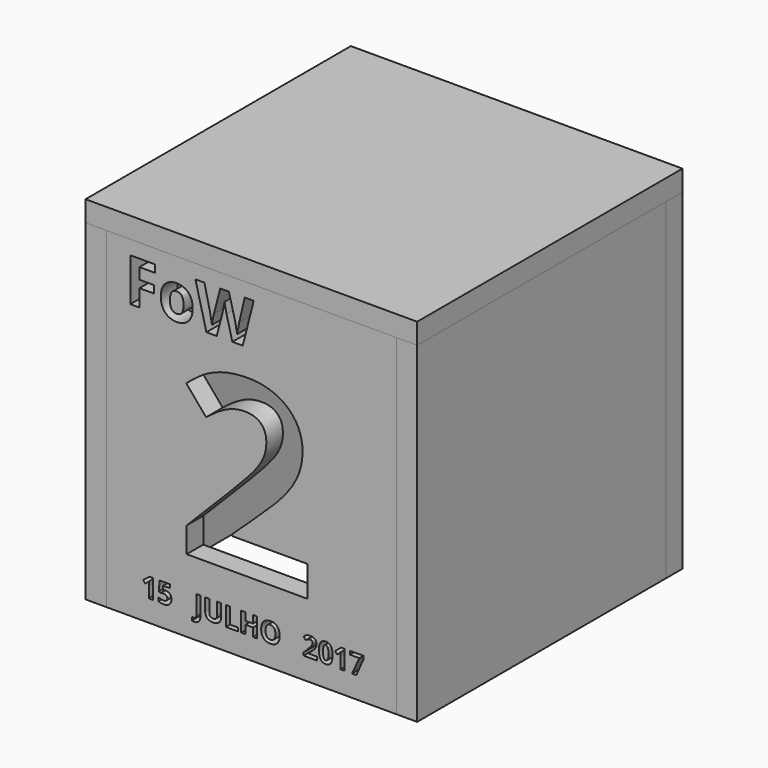
from build123d import *

# Parameters (mm, degrees)
F0_W            = 40
F0_H            = 40
F1_DEPTH        = 2.5
F2_W            = 40
F2_H            = 40
F3_DEPTH        = 2.5
F4_W            = 40
F4_H            = 40
F5_DEPTH        = 2.5
F6_W            = 40
F6_H            = 40
F7_DEPTH        = 2.5
F8_W            = 40
F8_H            = 40
F9_DEPTH        = 2.5
F10_TEXT_SIZE   = 7.2732438383
F10_TEXT_SIZE_2 = 29.1666666667
F10_TEXT_SIZE_3 = 3.2806804374
F11_DEPTH       = 3


# Not quite as in the source:
# - Text() gives the source's letters only with a copy of the font that has no kerning and outlines rounded to 1/6400 em; it was checked with that copy


with BuildPart() as f1:
    # F0 (on Top) → F1 (new body)
    with BuildSketch(Plane.XY):
        with Locations((-20, 20)):
            Rectangle(F0_W, F0_H)
    extrude(amount=F1_DEPTH)


with BuildPart() as f3:
    # F2 (on face) → F3 (new body)
    with BuildSketch(Plane.XZ):
        with Locations((-20, -20)):
            Rectangle(F2_W, F2_H)
    extrude(amount=-F3_DEPTH)

    # F10 (on face) → F11 (cut)
    with BuildSketch(Plane.XZ):
        with Locations((-35.2436941774, -6.8869412126)):
            Text('FoW', F10_TEXT_SIZE, font='Open Sans', font_style=FontStyle.BOLD, text_align=(TextAlign.LEFT, TextAlign.BOTTOM))
        with Locations((-28.9652795753, -31.2295894176)):
            Text('2', F10_TEXT_SIZE_2, font='Open Sans', font_style=FontStyle.BOLD, text_align=(TextAlign.LEFT, TextAlign.BOTTOM))
        with Locations((-33.2363452762, -37.4188534915)):
            Text('15   JULHO   2017', F10_TEXT_SIZE_3, font='Open Sans', font_style=FontStyle.BOLD, text_align=(TextAlign.LEFT, TextAlign.BOTTOM))
    extrude(amount=-F11_DEPTH, mode=Mode.SUBTRACT)


with BuildPart() as f5:
    # F4 (on face) → F5 (new body)
    with BuildSketch(Plane.YZ):
        with Locations((20, -20)):
            Rectangle(F4_W, F4_H)
    extrude(amount=-F5_DEPTH)


with BuildPart() as f7:
    # F6 (on face) → F7 (new body)
    with BuildSketch(Plane(origin=(0, 40, 0), x_dir=(-1, 0, 0), z_dir=(0, 1, 0))):
        with Locations((20, -20)):
            Rectangle(F6_W, F6_H)
    extrude(amount=-F7_DEPTH)


with BuildPart() as f9:
    # F8 (on face) → F9 (new body)
    with BuildSketch(Plane(origin=(-40, 0, 0), x_dir=(0, -1, 0), z_dir=(-1, 0, 0))):
        with Locations((-20, -20)):
            Rectangle(F8_W, F8_H)
    extrude(amount=-F9_DEPTH)


solid = Compound([f1.part, f3.part, f5.part, f7.part, f9.part])
